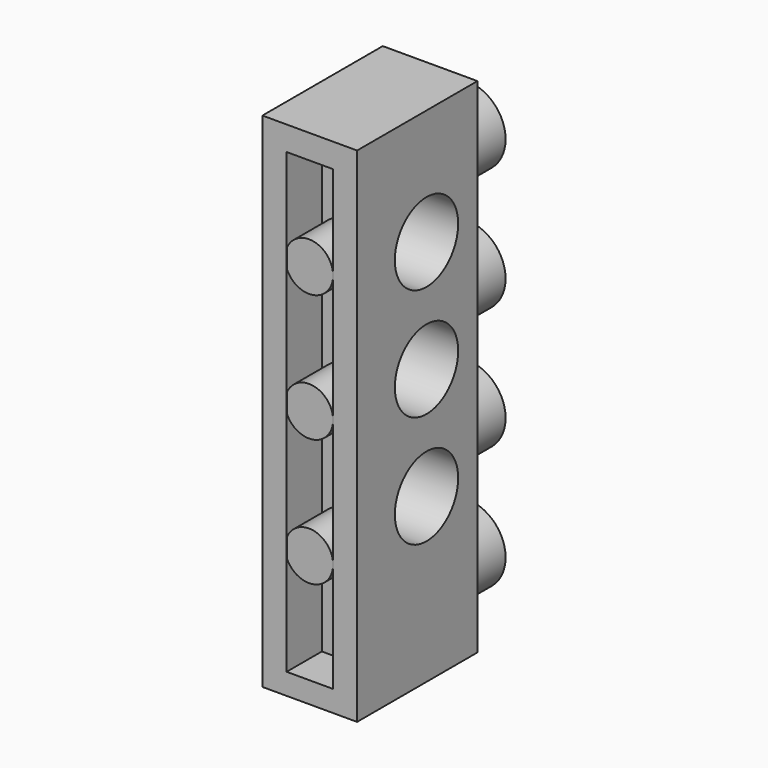
from build123d import *

# Parameters (mm, degrees)
F0_W     = 5.98
F0_H     = 31.77
F1_DEPTH = 9.5
F3_D     = 5
F4_R     = 2.445
F5_DEPTH = 2.69
F6_W     = 2.92
F6_H     = 28.9
F7_DEPTH = 2.78
F9_DEPTH = 2.75


with BuildPart() as f1:
    # F0 (on Front) → F1 (new body)
    with BuildSketch(Plane.XZ):
        with Locations((-21.5895947321, 10.6426752984)):
            Rectangle(F0_W, F0_H)
    extrude(amount=F1_DEPTH)

    # F3 (through all)
    with Locations(Plane.YZ):
        with Locations((-4.02, 19.2140168432), (-4.02, 12.1440168432), (-4.02, 5.0740168432)):
            Hole(F3_D / 2)

    # F4 (on Front) → F5 (join)
    with BuildSketch(Plane.XZ):
        with Locations((-21.4179256038, 22.0790577062)):
            Circle(F4_R)
        with Locations((-21.4179256038, 14.3290577062)):
            Circle(F4_R)
        with Locations((-21.4179256038, 6.5790577062)):
            Circle(F4_R)
        with Locations((-21.4179256038, -1.1709422938)):
            Circle(F4_R)
    extrude(amount=-F5_DEPTH)

    # F6 (on face) → F7 (cut)
    with BuildSketch(Plane.XZ.offset(9.5)):
        with Locations((-21.5895947321, 10.5476752984)):
            Rectangle(F6_W, F6_H)
    extrude(amount=-F7_DEPTH, mode=Mode.SUBTRACT)

    # F8 (on face) → F9 (join)
    with BuildSketch(Plane.XZ.offset(6.72)):
        with BuildLine():
            ThreePointArc((-23.0495947321, 18.4560718795), (-21.345700419, 17.5789010333), (-20.1375805098, 19.0665605403))
            ThreePointArc((-20.1375805098, 19.0665605403), (-21.345700419, 20.5542200474), (-23.0495947321, 19.6770492011))
            Line((-23.0495947321, 19.6770492011), (-23.0495947321, 18.4560718795))
        make_face()
        with BuildLine():
            ThreePointArc((-20.1375805098, 11.0265605403), (-21.345700419, 12.5142200474), (-23.0495947321, 11.6370492011))
            Line((-23.0495947321, 11.6370492011), (-23.0495947321, 10.4160718795))
            ThreePointArc((-23.0495947321, 10.4160718795), (-21.345700419, 9.5389010333), (-20.1375805098, 11.0265605403))
        make_face()
        with BuildLine():
            Line((-23.0495947321, 2.3760718795), (-23.0495947321, 3.5970492011))
            ThreePointArc((-23.0495947321, 3.5970492011), (-23.1775805098, 2.9865605403), (-23.0495947321, 2.3760718795))
        make_face()
        with BuildLine():
            ThreePointArc((-20.1375805098, 2.9865605403), (-21.345700419, 4.4742200474), (-23.0495947321, 3.5970492011))
            Line((-23.0495947321, 3.5970492011), (-23.0495947321, 2.3760718795))
            ThreePointArc((-23.0495947321, 2.3760718795), (-21.345700419, 1.4989010333), (-20.1375805098, 2.9865605403))
        make_face()
    extrude(amount=F9_DEPTH)


solid = f1.part
